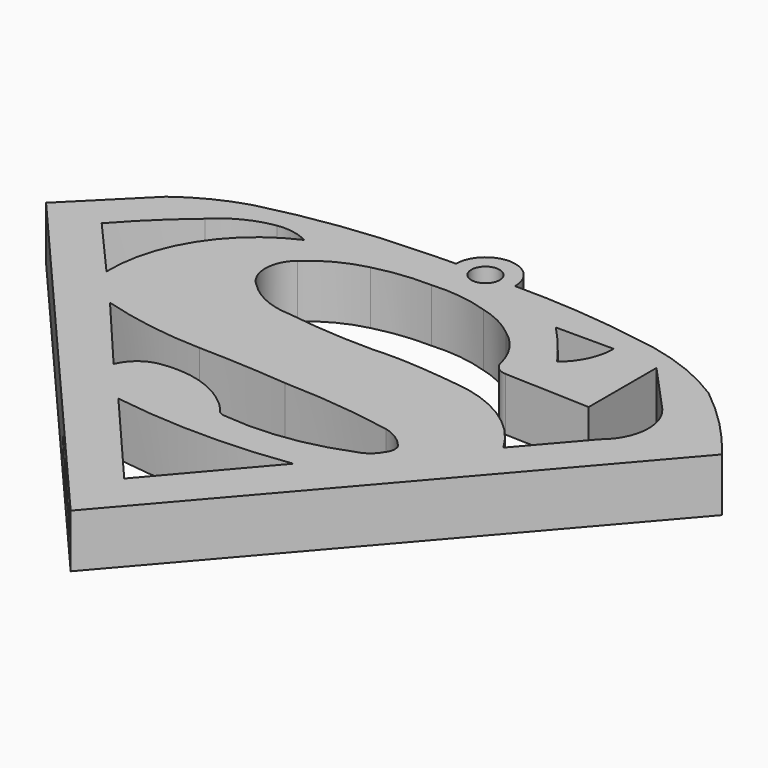
from build123d import *

# Parameters (mm, degrees)
F1_DEPTH     = 5
F2_TEXT_SIZE = 3.4640286079
F3_DEPTH     = 2


# Not quite as in the source:
# - Text() gives the source's letters only with a copy of the font that has no kerning and outlines rounded to 1/6400 em; it was checked with that copy


with BuildPart() as f1:
    # F0 (on Top) → F1 (new body)
    with BuildSketch(Plane.XY):
        with BuildLine():
            Line((7.4367700145, 44.008154422), (1.2063120957, 37.7950817347))
            Line((1.2063120957, 37.7950817347), (33.0417379737, 0.874263118))
            Line((33.0417379737, 0.874263118), (64.6454691887, 37.5447645783))
            ThreePointArc((64.6454691887, 37.5447645783), (61.4489252674, 41.2433511607), (57.8174330294, 44.5159189403))
            ThreePointArc((57.8174330294, 44.5159189403), (53.2299621564, 46.7747942089), (48.2485629618, 47.929380089))
            ThreePointArc((48.2485629618, 47.929380089), (42.2457288164, 48.6718824934), (36.2014225686, 48.8992359209))
            ThreePointArc((36.2014225686, 48.8992359209), (33.4441258395, 51.7298394679), (30.6136988617, 48.9723614869))
            ThreePointArc((30.6136988617, 48.9723614869), (28.9934443941, 48.9434336707), (27.3742617189, 48.8777920468))
            ThreePointArc((27.3742617189, 48.8777920468), (20.2356761184, 48.3110555564), (13.2069410756, 46.940844506))
            ThreePointArc((13.2069410756, 46.940844506), (10.1896547823, 45.7346091222), (7.4367700145, 44.008154422))
        make_face()
        with BuildLine():
            Line((32.926440239, 7.2841905057), (24.6811825782, 16.9049222022))
            ThreePointArc((24.6811825782, 16.9049222022), (32.8899726319, 16.2752961008), (41.1036945879, 16.836931929))
            Line((41.1036945879, 16.836931929), (32.926440239, 7.2841905057))
        make_face(mode=Mode.SUBTRACT)
        with BuildLine():
            Line((20.9998898208, 20.951975137), (14.7305028513, 28.3656641841))
            ThreePointArc((14.7305028513, 28.3656641841), (19.4579839087, 27.3005146226), (24.2848005146, 26.8698614091))
            ThreePointArc((24.2848005146, 26.8698614091), (28.4709953528, 26.7258024272), (32.6490625739, 26.4279190451))
            ThreePointArc((32.6490625739, 26.4279190451), (37.8326934355, 26.1045144086), (42.9723113775, 25.3568869084))
            ThreePointArc((42.9723113775, 25.3568869084), (44.3065893688, 24.7536793065), (45.3654639423, 23.7422734499))
            ThreePointArc((45.3654639423, 23.7422734499), (45.4533072794, 23.0533432204), (45.1531857252, 22.4270299077))
            ThreePointArc((45.1531857252, 22.4270299077), (44.5114706688, 21.6452658759), (43.616682291, 21.1737714708))
            ThreePointArc((43.616682291, 21.1737714708), (38.1415944776, 19.7058568795), (32.4737913907, 19.6200199425))
            ThreePointArc((32.4737913907, 19.6200199425), (31.9467232322, 19.7889408885), (31.5594412386, 20.1843492687))
            ThreePointArc((31.5594412386, 20.1843492687), (31.2128748249, 20.5877457791), (30.8253519241, 20.951975137))
            ThreePointArc((30.8253519241, 20.951975137), (27.4130625136, 22.8509308738), (23.5132284618, 23.0535296874))
            ThreePointArc((23.5132284618, 23.0535296874), (21.991186024, 22.3201234316), (20.9998898208, 20.951975137))
        make_face(mode=Mode.SUBTRACT)
        with BuildLine():
            ThreePointArc((16.6400652379, 45.5157384276), (18.1667662697, 45.4823270871), (19.6079816669, 44.9775196612))
            ThreePointArc((19.6079816669, 44.9775196612), (13.5789128466, 39.7494821025), (11.4477267489, 32.0592224598))
            Line((11.4477267489, 32.0592224598), (6.4057447016, 37.7987548709))
            ThreePointArc((6.4057447016, 37.7987548709), (9.0244475118, 40.5380787665), (11.8459155783, 43.0680625141))
            ThreePointArc((11.8459155783, 43.0680625141), (14.0460179451, 44.6777013284), (16.6400652379, 45.5157384276))
        make_face(mode=Mode.SUBTRACT)
        with BuildLine():
            Line((56.1948753893, 33.8508561254), (51.5019446611, 28.412014246))
            ThreePointArc((51.5019446611, 28.412014246), (47.6483472605, 32.3935209591), (42.391397059, 34.1448299587))
            ThreePointArc((42.391397059, 34.1448299587), (40.1110001019, 34.3994865891), (37.8233455122, 34.5775224268))
            ThreePointArc((37.8233455122, 34.5775224268), (36.0637735575, 34.6255168358), (34.3042016029, 34.5775224268))
            ThreePointArc((34.3042016029, 34.5775224268), (30.1882894184, 34.7131240055), (26.0940790176, 35.1564772427))
            ThreePointArc((26.0940790176, 35.1564772427), (23.5783294526, 35.7080405232), (21.4415397495, 37.1458679438))
            ThreePointArc((21.4415397495, 37.1458679438), (20.2001771957, 39.5841648143), (21.2798025459, 42.098261416))
            ThreePointArc((21.2798025459, 42.098261416), (23.5285899932, 43.660937108), (26.0940790176, 44.6186773479))
            ThreePointArc((26.0940790176, 44.6186773479), (28.6889342817, 45.1040979638), (31.3263013959, 45.2189967036))
            ThreePointArc((31.3263013959, 45.2189967036), (34.0456159578, 45.14962183), (36.7014780641, 44.5615053177))
            ThreePointArc((36.7014780641, 44.5615053177), (38.5694970602, 43.8717602708), (40.2416177094, 42.7904389799))
            ThreePointArc((40.2416177094, 42.7904389799), (41.9985313234, 41.0005323758), (43.0064946413, 38.7038998306))
            ThreePointArc((43.0064946413, 38.7038998306), (43.4863938344, 37.9414531109), (44.3288236856, 37.6221723855))
            Line((44.3288236856, 37.6221723855), (52.3589812219, 37.3096689582))
            Line((52.3589812219, 37.3096689582), (52.3589812219, 45.2423617244))
            Line((52.3589812219, 45.2423617244), (56.7691959441, 40.4190085828))
            ThreePointArc((56.7691959441, 40.4190085828), (57.8681050316, 37.0137341737), (56.1948753893, 33.8508561254))
        make_face(mode=Mode.SUBTRACT)
        with BuildLine():
            ThreePointArc((46.078088152, 41.4777850025), (44.4169489146, 43.6212921153), (42.6213517785, 45.6534922123))
            Line((42.6213517785, 45.6534922123), (48.0421964597, 45.6534922123))
            ThreePointArc((48.0421964597, 45.6534922123), (47.5266544217, 43.3462074365), (46.078088152, 41.4777850025))
        make_face(mode=Mode.SUBTRACT)
        with BuildLine():
            ThreePointArc((34.7270810555, 48.8807908197), (32.0871799289, 48.9635770306), (34.7282346021, 48.9359776087))
            ThreePointArc((34.7282346021, 48.9359776087), (34.727946184, 48.9083781869), (34.7270810555, 48.8807908197))
        make_face(mode=Mode.SUBTRACT)
    extrude(amount=F1_DEPTH)

    # F2 (on face) → F3 (cut)
    with BuildSketch(Plane(origin=(19.3838015142, 16.7139191236, 0), x_dir=(0.6530235662, -0.7573375878, 0), z_dir=(-0.7573375878, -0.6530235662, 0))):
        with Locations((4.9496158026, 1.1457368964)):
            Text('ADRIANA', F2_TEXT_SIZE, font='Open Sans', text_align=(TextAlign.LEFT, TextAlign.BOTTOM))
    extrude(amount=-F3_DEPTH, mode=Mode.SUBTRACT)


solid = f1.part
